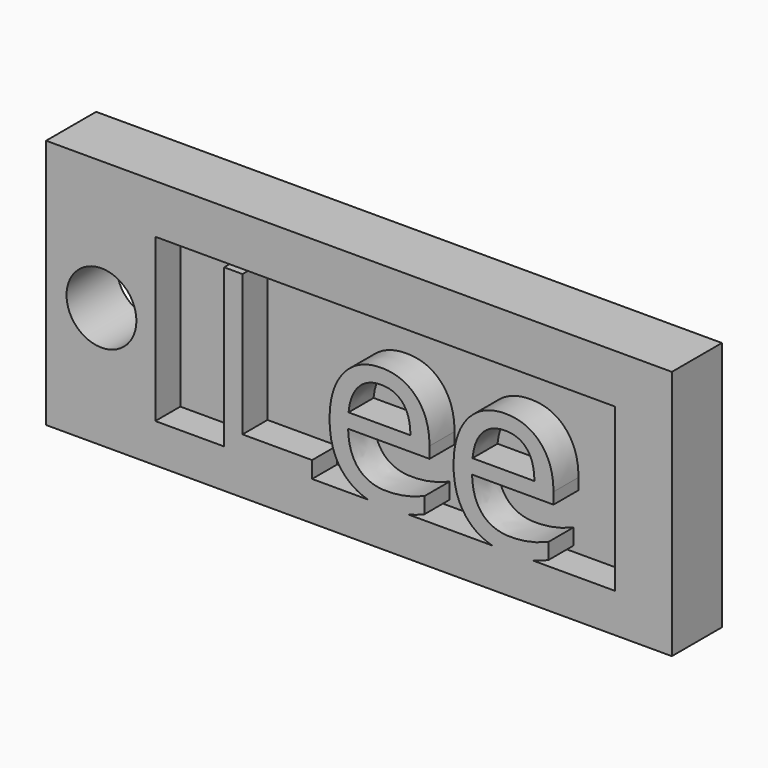
from build123d import *

# Parameters (mm, degrees)
F0_W         = 63.5
F0_H         = 25.4
F0_W_2       = 46.6525433585
F0_H_2       = 16.4656043053
F1_DEPTH     = 6.35
F2_DEPTH     = 3.175
F3_R         = 3.5456892192
F4_DEPTH     = 25.4
F5_TEXT_SIZE = 22.4199015333
F6_DEPTH     = 3.175


# Not quite as in the source:
# - Text() gives the source's letters only with a copy of the font that has no kerning and outlines rounded to 1/6400 em; it was checked with that copy


with BuildPart() as f1:
    # F0 (on Front) → F1 (new body)
    with BuildSketch(Plane.XZ):
        with Locations((31.75, 12.7)):
            Rectangle(F0_W, F0_H)
        with Locations((34.4082550146, 12.1932607144)):
            Rectangle(F0_W_2, F0_H_2, mode=Mode.SUBTRACT)
    extrude(amount=F1_DEPTH)

    # F0 (on Front) → F2 (join)
    with BuildSketch(Plane.XZ):
        with Locations((34.4082550146, 12.1932607144)):
            Rectangle(F0_W_2, F0_H_2)
    extrude(amount=F2_DEPTH)

    # F3 (on face) → F4 (cut)
    with BuildSketch(Plane.XZ.offset(6.35)):
        with Locations((5.6201964617, 12.2865745798)):
            Circle(F3_R)
    extrude(amount=-F4_DEPTH, mode=Mode.SUBTRACT)

    # F5 (on face) → F6 (join)
    with BuildSketch(Plane.XZ.offset(3.175)):
        with Locations((15.8697989342, 3.9604585618)):
            Text('Lee', F5_TEXT_SIZE, font='Open Sans', text_align=(TextAlign.LEFT, TextAlign.BOTTOM))
    extrude(amount=F6_DEPTH)


solid = f1.part
